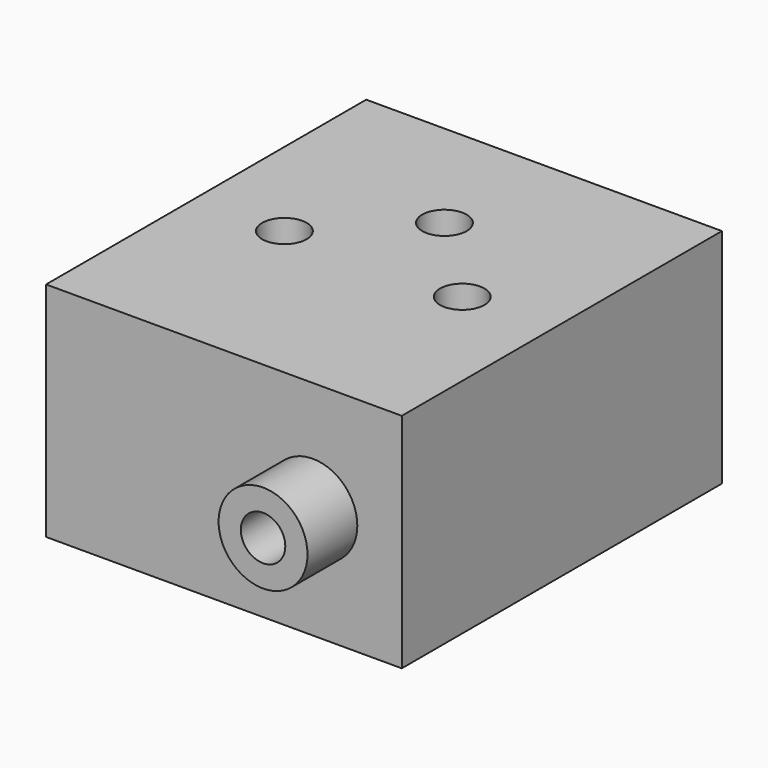
from build123d import *

# Parameters (mm, degrees)
F0_W          = 40
F0_H          = 25
F1_DEPTH      = 45
F2_R          = 5
F3_DEPTH      = 7
F4_R          = 2.5
F5_DEPTH      = 45.001
F5_DEPTH_BACK = 7.001
F6_R          = 2.5
F7_DEPTH      = 25.001


with BuildPart() as f1:
    # F0 (on Front) → F1 (new body)
    with BuildSketch(Plane.XZ):
        with Locations((-10, 0)):
            Rectangle(F0_W, F0_H)
    extrude(amount=-F1_DEPTH)

    # F2 (on face) → F3 (join)
    with BuildSketch(Plane.XZ):
        Circle(F2_R)
    extrude(amount=F3_DEPTH)

    # F4 (on Front) → F5 (cut, two sides)
    with BuildSketch(Plane.XZ) as f5_sk:
        Circle(F4_R)
    extrude(amount=-F5_DEPTH, mode=Mode.SUBTRACT)
    extrude(f5_sk.sketch, amount=F5_DEPTH_BACK, mode=Mode.SUBTRACT)

    # F6 (on face) → F7 (cut, through all)
    with BuildSketch(Plane.XY.offset(12.5)):
        with Locations((0, 21)):
            Circle(F6_R)
        with Locations((-10, 31)):
            Circle(F6_R)
        with Locations((-20, 21)):
            Circle(F6_R)
    extrude(amount=-F7_DEPTH, mode=Mode.SUBTRACT)


solid = f1.part
